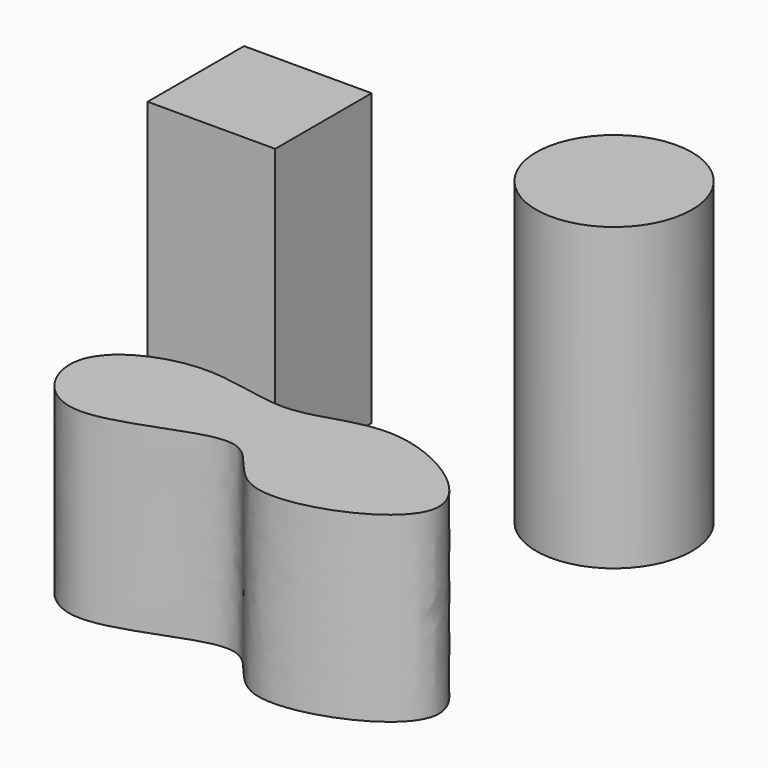
from build123d import *

# Parameters (mm, degrees)
F1_DEPTH = 54
F0_R     = 23.0555619828
F2_DEPTH = 89
F0_W     = 37.7743057907
F0_H     = 35.6949903071
F3_DEPTH = 86


# Not quite as in the source:
# - the program builds the solid bodies; features that only make, move or delete a surface that nothing else refers to are left out


with BuildPart() as f1:
    # F0 (on Top) → F1 (new body)
    with BuildSketch(Plane.XY):
        with BuildLine():
            add(Edge.make_bspline(
                [(-39.8536287248, -27.7242679149), (-50.2375219072, -28.2925626406), (-72.053468967, -38.4287091274), (-52.3114138524, -73.8395869052), (-5.4344000682, -40.8979144482), (2.0226294599, -77.3246249013), (67.3517685782, -51.0572269021), (16.3081275338, -17.8312624321), (-9.7598597024, -35.967977136), (-29.1378204925, -27.1378079818), (-39.8536287248, -27.7242679149)],
                knots=[0, 0, 0, 0, 0.1177566126, 0.2265475614, 0.3710310856, 0.4768512147, 0.6224209007, 0.7571839019, 0.8784793664, 1, 1, 1, 1], degree=3))
        make_face()
    extrude(amount=F1_DEPTH)


with BuildPart() as f2:
    # F0 (on Top) → F2 (new body)
    with BuildSketch(Plane.XY):
        with Locations((18.7138784677, 52.6760928333)):
            Circle(F0_R)
    extrude(amount=F2_DEPTH)


with BuildPart() as f3:
    # F0 (on Top) → F3 (new body)
    with BuildSketch(Plane.XY):
        with Locations((-75.0287864357, 38.6406872422)):
            Rectangle(F0_W, F0_H)
    extrude(amount=F3_DEPTH)


solid = Compound([f1.part, f2.part, f3.part])
